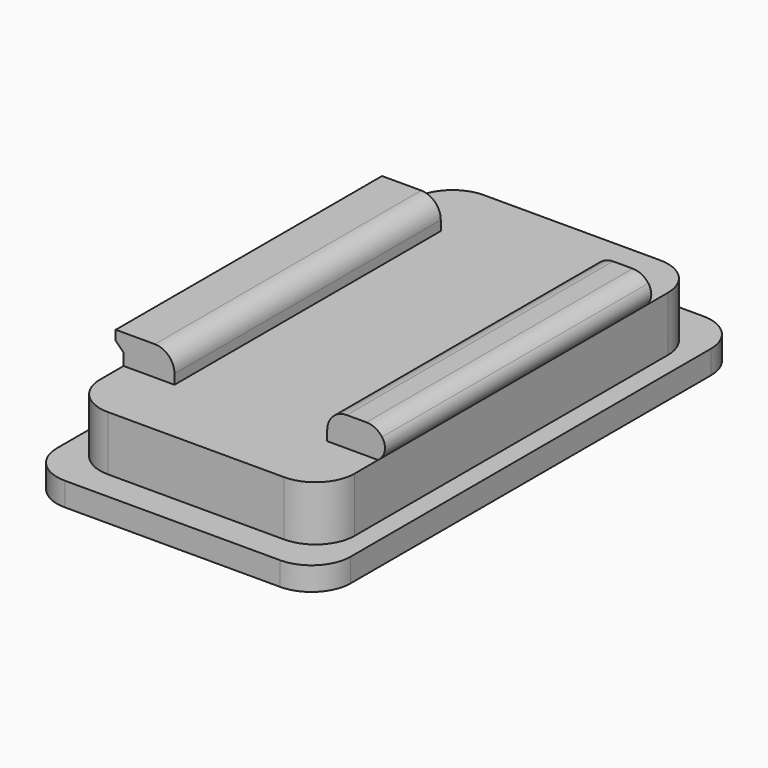
from build123d import *

# Parameters (mm, degrees)
F0_W        = 15
F0_H        = 27
F0_W_2      = 13
F0_H_2      = 24
F1_DEPTH    = 1.2
F2_DEPTH    = 4
F3_R        = 2
F4_W        = 2.6
F4_H        = 17
F4_W_2      = 0.4
F5_DEPTH    = 1.5
F6_T1_DEPTH = 21
F6_T3_DEPTH = 22
F7_T4_DEPTH = 22.1433659759
F8_R        = 0.75


# Not quite as in the source:
# - a fillet or chamfer that OpenCascade refuses, or shapes differently, is made with other operations: its cross-section is extruded or revolved along the edge and cut away or added


with BuildPart() as f1:
    # F0 (on Top) → F1 (new body)
    with BuildSketch(Plane.XY):
        Rectangle(F0_W, F0_H)
        Rectangle(F0_W_2, F0_H_2, mode=Mode.SUBTRACT)
    extrude(amount=F1_DEPTH)

    # F0 (on Top) → F2 (join)
    with BuildSketch(Plane.XY):
        Rectangle(F0_W_2, F0_H_2)
    extrude(amount=F2_DEPTH)

    # F3
    f3_edges = [f1.edges().sort_by_distance(p)[0] for p in [
        (6.5, 12, 2.6),
        (7.5, 13.5, 0.6),
        (-6.5, 12, 2.6),
        (-7.5, 13.5, 0.6),
        (-6.5, -12, 2.6),
        (-7.5, -13.5, 0.6),
        (7.5, -13.5, 0.6),
        (6.5, -12, 2.6),
    ]]
    fillet(f3_edges, radius=F3_R)

    # F4 (on face) → F5 (join)
    with BuildSketch(Plane.XY.offset(4)):
        with Locations((-5.2, 0)):
            Rectangle(F4_W, F4_H)
        with Locations((6.7, 0)):
            Rectangle(F4_W_2, F4_H)
        with Locations((5.2, 0)):
            Rectangle(F4_W, F4_H)
        with Locations((-6.7, 0)):
            Rectangle(F4_W_2, F4_H)
    extrude(amount=F5_DEPTH)

    # F6: fillet of radius 1 on 4 edges, made by hand

    # F6_s2 → F6_t1 (cut)
    with BuildSketch(Plane.XZ.offset(-10.5)):
        with BuildLine():
            ThreePointArc((6.5, 4), (6.794427191, 4.3527864045), (6.9, 4.8))
            Line((6.9, 4.8), (6.9, 4))
            Line((6.9, 4), (6.5, 4))
        make_face()
    extrude(amount=F6_T1_DEPTH, mode=Mode.SUBTRACT)

    # F6_s4 → F6_t3 (cut)
    with BuildSketch(Plane.XZ.offset(-11)):
        with BuildLine():
            ThreePointArc((6.9, 4.5), (6.6071067812, 5.2071067812), (5.9, 5.5))
            Line((5.9, 5.5), (6.9, 5.5))
            Line((6.9, 5.5), (6.9, 4.5))
        make_face()
        with BuildLine():
            ThreePointArc((-3.9, 4.5), (-4.1928932188, 5.2071067812), (-4.9, 5.5))
            Line((-4.9, 5.5), (-3.9, 5.5))
            Line((-3.9, 5.5), (-3.9, 4.5))
        make_face()
        with BuildLine():
            ThreePointArc((3.9, 4.5), (4.1928932188, 5.2071067812), (4.9, 5.5))
            Line((4.9, 5.5), (3.9, 5.5))
            Line((3.9, 5.5), (3.9, 4.5))
        make_face()
    extrude(amount=F6_T3_DEPTH, mode=Mode.SUBTRACT)

    # F7: chamfer of 1 on 1 edges, made by hand


with BuildPart() as f7_tool2:
    # F7_s3 → F7_t4 (new body)
    with BuildSketch(Plane.XZ.offset(-11.071682988)):
        Polygon((-5.9, 4), (-6.9, 5), (-6.9, 4), align=None)
    extrude(amount=F7_T4_DEPTH)

    split(bisect_by=Plane.YZ.offset(-6.5), keep=Keep.BOTTOM)


with BuildPart() as f1_1:
    add(f1.part)

    # F7_t1: cut F7_tool2
    add(f7_tool2.part, mode=Mode.SUBTRACT)

    # F8
    f8_edges = [f1_1.edges().sort_by_distance(p)[0] for p in [
        (6.888686, 0, 4.65),
    ]]
    fillet(f8_edges, radius=F8_R)


solid = f1_1.part
